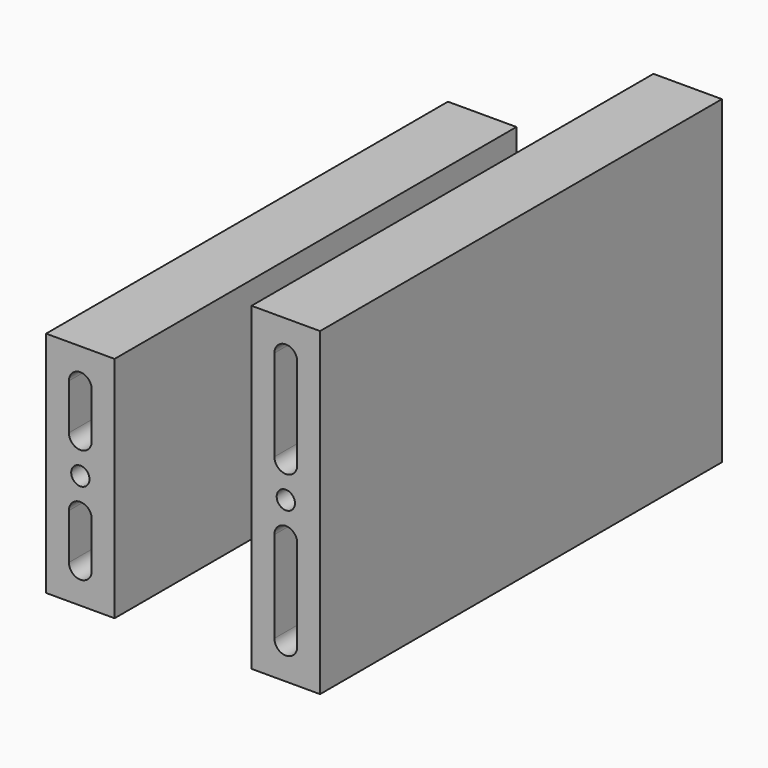
from build123d import *
from build123d import SkipClean  # not in build123d's __all__

# Parameters (mm, degrees)
F0_W      = 38.1
F0_H      = 127
F0_R      = 5.08
F1_DEPTH  = 25.4
F0_H_2    = 177.8
F2_W      = 38.1
F2_H      = 177.8
F3_DEPTH  = 254
F2_H_2    = 127
F4_R      = 5.08
F5_DEPTH  = 63.5
F6_R      = 15.875
F7_DEPTH  = 28.575
F10_W     = 2.0828
F10_H     = 7.9375
F12_R     = 4.7625
F13_DEPTH = 8.334375


with BuildPart() as f1:
    # F0 (on Front) → F1 (new body)
    with BuildSketch(Plane.XZ):
        with Locations((-19.05, 63.5)):
            Rectangle(F0_W, F0_H)
        with BuildLine():
            Line((-25.4, 19.05), (-25.4, 44.45))
            ThreePointArc((-25.4, 44.45), (-19.05, 50.8), (-12.7, 44.45))
            Line((-12.7, 44.45), (-12.7, 19.05))
            ThreePointArc((-12.7, 19.05), (-19.05, 12.7), (-25.4, 19.05))
        make_face(mode=Mode.SUBTRACT)
        with Locations((-19.05, 63.5)):
            Circle(F0_R, mode=Mode.SUBTRACT)
        with BuildLine():
            Line((-12.7, 107.95), (-12.7, 82.55))
            ThreePointArc((-12.7, 82.55), (-19.05, 76.2), (-25.4, 82.55))
            Line((-25.4, 82.55), (-25.4, 107.95))
            ThreePointArc((-25.4, 107.95), (-19.05, 114.3), (-12.7, 107.95))
        make_face(mode=Mode.SUBTRACT)
    extrude(amount=F1_DEPTH)

    # F2 (on face) → F3, piece 2 (join)
    with BuildSketch(Plane(origin=(0, 0, 0), x_dir=(-1, 0, 0), z_dir=(0, 1, 0))):
        with Locations((19.05, 63.5)):
            Rectangle(F2_W, F2_H_2)
    extrude(amount=F3_DEPTH)


with BuildPart() as f1b:
    # F0 (on Front) → F1, piece 2 (new body)
    with BuildSketch(Plane.XZ):
        with Locations((95.25, 88.9)):
            Rectangle(F0_W, F0_H_2)
        with BuildLine():
            Line((101.6, 69.85), (101.6, 19.05))
            ThreePointArc((101.6, 19.05), (95.25, 12.7), (88.9, 19.05))
            Line((88.9, 19.05), (88.9, 69.85))
            ThreePointArc((88.9, 69.85), (95.25, 76.2), (101.6, 69.85))
        make_face(mode=Mode.SUBTRACT)
        with Locations((95.25, 88.9)):
            Circle(F0_R, mode=Mode.SUBTRACT)
        with BuildLine():
            ThreePointArc((101.6, 107.95), (95.25, 101.6), (88.9, 107.95))
            Line((88.9, 107.95), (88.9, 158.75))
            ThreePointArc((88.9, 158.75), (95.25, 165.1), (101.6, 158.75))
            Line((101.6, 158.75), (101.6, 107.95))
        make_face(mode=Mode.SUBTRACT)
    extrude(amount=F1_DEPTH)

    # F2 (on face) → F3 (join)
    with BuildSketch(Plane(origin=(0, 0, 0), x_dir=(-1, 0, 0), z_dir=(0, 1, 0))):
        with Locations((-95.25, 88.9)):
            Rectangle(F2_W, F2_H)
    extrude(amount=F3_DEPTH)


with BuildPart() as f5_tool:
    # F4 (on face) → F5 (new body)
    with BuildSketch(Plane.XZ):
        with Locations((-19.05, 63.5)):
            Circle(F4_R)
        with Locations((95.25, 88.9)):
            Circle(F4_R)
    extrude(amount=-F5_DEPTH)


with BuildPart() as f1_1:
    add(f1.part, clean=False)

    # F5: cut by f5_tool
    add(f5_tool.part, mode=Mode.SUBTRACT)

    # F6 (on face) → F7 (cut)
    with BuildSketch(Plane(origin=(-38.1, 0, 0), x_dir=(0, -1, 0), z_dir=(-1, 0, 0))):
        with Locations((-38.1, 63.5)):
            Circle(F6_R)
    extrude(amount=-F7_DEPTH, mode=Mode.SUBTRACT)


with BuildPart() as f1b_1:
    add(f1b.part, clean=False)

    # F5: cut by f5_tool
    add(f5_tool.part, mode=Mode.SUBTRACT)


with BuildPart() as f11:
    # F10 (on plane+point) → F11 (revolve)
    with BuildSketch(Plane(origin=(-19.05, 0, 0), x_dir=(0, -1, 0), z_dir=(-1, 0, 0))):
        with Locations((-29.6164, 72.23125)):
            Rectangle(F10_W, F10_H)
    revolve(axis=Axis((-19.05, 9.597724928, 63.5), (0, -1, 0)))

    # F12 (on face) → F13 (join)
    with BuildSketch(Plane(origin=(0, 30.6578, 0), x_dir=(-1, 0, 0), z_dir=(0, 1, 0))):
        Polygon((27.298891971, 63.5), (23.1744459855, 70.64375), (14.9255540145, 70.64375), (10.801108029, 63.5), (14.9255540145, 56.35625), (23.1744459855, 56.35625), align=None)
        with Locations((19.05, 63.5)):
            Circle(F12_R, mode=Mode.SUBTRACT)
    with SkipClean():  # cleaning this boolean's faces spoils the solid; the shape is the same uncleaned
        extrude(amount=F13_DEPTH)


solid = Compound([f1_1.part, f1b_1.part, f11.part])
